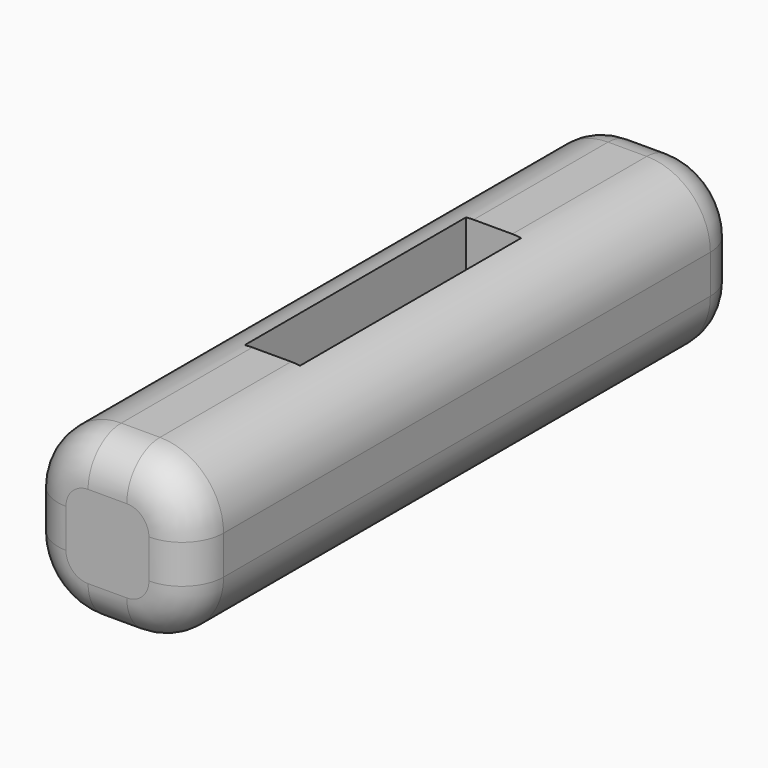
from build123d import *

# Parameters (mm, degrees)
F0_W        = 6
F0_H        = 25
F0_W_2      = 2
F0_H_2      = 10
F1_DEPTH    = 6
F2_T1_DEPTH = 36.5
F3_R        = 1.5


# Not quite as in the source:
# - a fillet or chamfer that OpenCascade refuses, or shapes differently, is made with other operations: its cross-section is extruded or revolved along the edge and cut away or added


with BuildPart() as f1:
    # F0 (on Top) → F1 (new body)
    with BuildSketch(Plane.XY):
        with Locations((-10.7731075219, -2.0936969668)):
            Rectangle(F0_W, F0_H)
        with Locations((-10.7510519922, -2.1686129086)):
            Rectangle(F0_W_2, F0_H_2, mode=Mode.SUBTRACT)
    extrude(amount=F1_DEPTH)

    # F2: fillet of radius 2.3 on 4 edges, made by hand

    # F2_s2 → F2_t1 (cut)
    with BuildSketch(Plane.XZ.offset(-16.1563030332)):
        with BuildLine():
            ThreePointArc((-13.7731075219, 3.7), (-13.0994531186, 5.3263455967), (-11.4731075219, 6))
            Line((-11.4731075219, 6), (-13.7731075219, 6))
            Line((-13.7731075219, 6), (-13.7731075219, 3.7))
        make_face()
        with BuildLine():
            ThreePointArc((-13.7731075219, 2.3), (-13.0994531186, 0.6736544033), (-11.4731075219, 0))
            Line((-11.4731075219, 0), (-13.7731075219, 0))
            Line((-13.7731075219, 0), (-13.7731075219, 2.3))
        make_face()
        with BuildLine():
            ThreePointArc((-7.7731075219, 3.7), (-8.4467619252, 5.3263455967), (-10.0731075219, 6))
            Line((-10.0731075219, 6), (-7.7731075219, 6))
            Line((-7.7731075219, 6), (-7.7731075219, 3.7))
        make_face()
        with BuildLine():
            ThreePointArc((-7.7731075219, 2.3), (-8.4467619252, 0.6736544033), (-10.0731075219, 0))
            Line((-10.0731075219, 0), (-7.7731075219, 0))
            Line((-7.7731075219, 0), (-7.7731075219, 2.3))
        make_face()
    extrude(amount=F2_T1_DEPTH, mode=Mode.SUBTRACT)

    # F3
    f3_edges = [f1.edges().sort_by_distance(p)[0] for p in [
        (-8.446762, 10.406303, 5.326346),
        (-10.773108, 10.406303, 6),
        (-13.099453, 10.406303, 5.326346),
        (-13.773108, 10.406303, 3),
        (-13.099453, 10.406303, 0.673654),
        (-8.446762, 10.406303, 0.673654),
        (-7.773108, 10.406303, 3),
        (-10.773108, 10.406303, 0),
        (-13.099453, -14.593697, 0.673654),
    ]]
    fillet(f3_edges, radius=F3_R)


solid = f1.part
